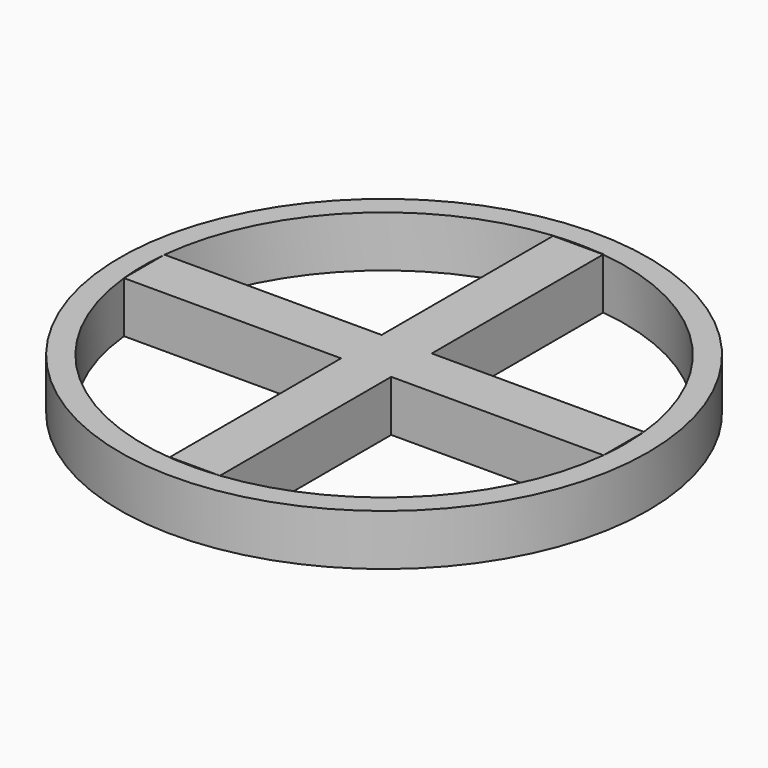
from build123d import *

# Parameters (mm, degrees)
F0_R     = 65.5602022546
F1_DEPTH = 12.7
F0_W     = 12.4544380459
F0_H     = 53.2347456641
F0_W_2   = 52.7194491877
F0_H_2   = 12.5804708937
F0_H_3   = 53.1745559146


with BuildPart() as f1:
    # F0 (on Top) → F1 (new body)
    with BuildSketch(Plane.XY):
        Circle(F0_R)
        with BuildLine():
            ThreePointArc((6.8319624097, 59.4948862362), (44.6959461159, 39.8571147906), (59.8858681045, 0))
            ThreePointArc((59.8858681045, 0), (59.802195524, -3.1645867238), (59.5514115975, -6.3203303216))
            ThreePointArc((59.5514115975, -6.3203303216), (42.5273022343, -42.1633224889), (6.8319624097, -59.4948862362))
            ThreePointArc((6.8319624097, -59.4948862362), (-37.4395303101, -46.7396915777), (-59.5514115975, -6.3203303216))
            Line((-59.5514115975, -6.3203303216), (-59.5577689193, -6.3203303216))
            Line((-59.5577689193, -6.3203303216), (-59.5577689193, -6.2601405721))
            ThreePointArc((-59.5577689193, -6.2601405721), (-59.8858681045, 0), (-59.5577689193, 6.2601405721))
            ThreePointArc((-59.5577689193, 6.2601405721), (-42.1185309141, 42.5716637244), (-5.6224756362, 59.621346566))
            ThreePointArc((-5.6224756362, 59.621346566), (0, 59.8858681045), (5.6224756362, 59.621346566))
            Line((5.6224756362, 59.621346566), (6.8319624097, 59.621346566))
            Line((6.8319624097, 59.621346566), (6.8319624097, 59.4948862362))
        make_face(mode=Mode.SUBTRACT)
    extrude(amount=F1_DEPTH)


with BuildPart() as f1b:
    # F0 (on Top) → F1, piece 2 (new body)
    with BuildSketch(Plane.XY):
        with Locations((0.6047433868, 32.8775134042)):
            Rectangle(F0_W, F0_H)
        with Locations((33.1916870036, -0.0300948747)):
            Rectangle(F0_W_2, F0_H_2)
        with Locations((0.6047433868, -0.0300948747)):
            Rectangle(F0_W, F0_H_2)
        with Locations((0.6047433868, -32.9076082789)):
            Rectangle(F0_W, F0_H_3)
        with BuildLine():
            Line((-5.6224756362, -6.3203303216), (-5.6224756362, 6.2601405721))
            Line((-5.6224756362, 6.2601405721), (-59.5577689193, 6.2601405721))
            Line((-59.5577689193, 6.2601405721), (-59.5577689193, -6.2601405721))
            ThreePointArc((-59.5577689193, -6.2601405721), (-59.5545978624, -6.29023625), (-59.5514115975, -6.3203303216))
            Line((-59.5514115975, -6.3203303216), (-5.6224756362, -6.3203303216))
        make_face()
    extrude(amount=F1_DEPTH)


solid = Compound([f1.part, f1b.part])
